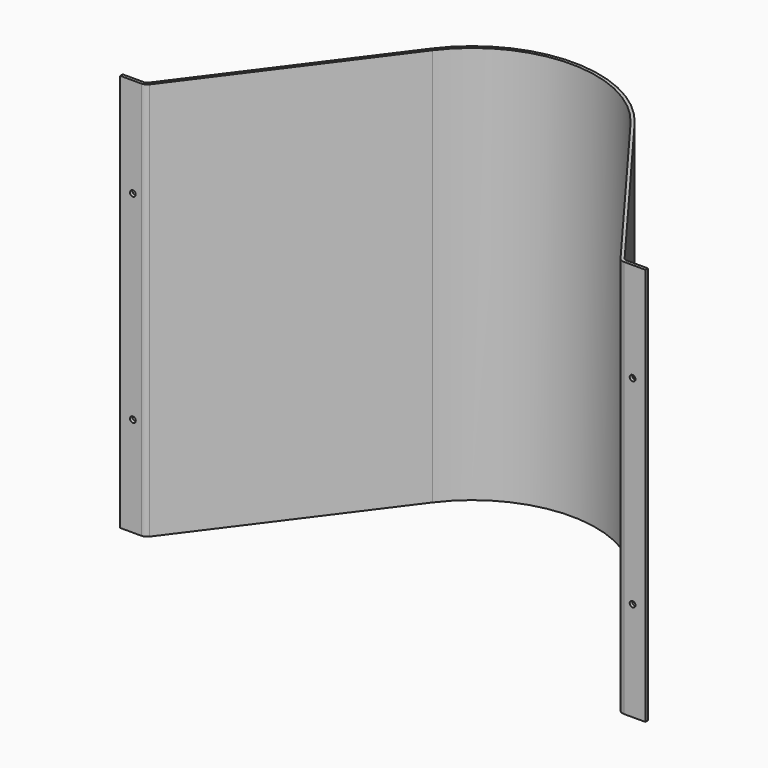
from build123d import *

# Parameters (mm, degrees)
F1_DEPTH = 609.6
F2_T     = 2.38125
F3_W     = 393.7
F3_H     = 155.575
F4_DEPTH = 179.0405708
F5_R     = 2.15265
F6_DEPTH = 2.38125


# Not quite as in the source:
# - a shell that OpenCascade refuses in one call is made with other operations: the cavity is built on its own and cut out


with BuildPart() as f1:
    # F0 (on Top) → F1 (new body)
    with BuildSketch(Plane.XY):
        with BuildLine():
            Line((15.875, 0), (0, 0))
            Line((0, 0), (0, -2.38125))
            Line((0, -2.38125), (393.7, -2.38125))
            Line((393.7, -2.38125), (393.7, 0))
            Line((393.7, 0), (377.825, 0))
            ThreePointArc((377.825, 0), (376.4007720387, 0.337360186), (375.2792072647, 1.2777482116))
            Line((375.2792072647, 1.2777482116), (273.096492423, 138.389761864))
            ThreePointArc((273.096492423, 138.389761864), (196.85, 176.6583208), (120.603507577, 138.389761864))
            Line((120.603507577, 138.389761864), (18.4207927353, 1.2777482116))
            ThreePointArc((18.4207927353, 1.2777482116), (17.2992279613, 0.337360186), (15.875, 0))
        make_face()
    extrude(amount=F1_DEPTH)

    # F2: shell of thickness 2.38125, made by hand


with BuildPart() as f2_core1:
    # F2_t2: copy of F1
    add(f1.part)

    # the walls: a layer under each face that stays
    f2_faces = [f2_core1.faces().sort_by_distance(p)[0] for p in [
        (196.85, 176.6583208, 304.8),
        (69.5121501562, 69.8337550378, 304.8),
        (17.2992279613, 0.337360186, 304.8),
        (7.9375, 0, 304.8),
        (0, -1.190625, 304.8),
        (393.7, -1.190625, 304.8),
        (385.7625, 0, 304.8),
        (376.4007720387, 0.337360186, 304.8),
        (324.1878498438, 69.8337550378, 304.8),
        (196.85, 87.1385354, 0),
        (196.85, 87.1385354, 609.6),
    ]]
    thicken(f2_faces, amount=-F2_T, mode=Mode.SUBTRACT)


with BuildPart() as f1_1:
    add(f1.part)

    # what is left inside the walls is the cavity
    f2_cavity = [f2_core1.part.solids().sort_by_distance(p)[0] for p in [
        (196.85, -2.357438, 405.60625),
    ]]
    add(f2_cavity, mode=Mode.SUBTRACT)

    # F3 (on face) → F4 (cut, through all)
    with BuildSketch(Plane.XZ.offset(2.38125)):
        with Locations((196.85, 531.8125)):
            Rectangle(F3_W, F3_H)
        with Locations((196.85, 77.7875)):
            Rectangle(F3_W, F3_H)
    extrude(amount=-F4_DEPTH, mode=Mode.SUBTRACT)

    # F5 (on face) → F6 (cut, through all)
    with BuildSketch(Plane.XZ.offset(2.38125)):
        with Locations((384.175, 230.1875)):
            Circle(F5_R)
        with Locations((384.175, 379.4125)):
            Circle(F5_R)
        with Locations((9.525, 379.4125)):
            Circle(F5_R)
        with Locations((9.525, 230.1875)):
            Circle(F5_R)
    extrude(amount=-F6_DEPTH, mode=Mode.SUBTRACT)


solid = f1_1.part
